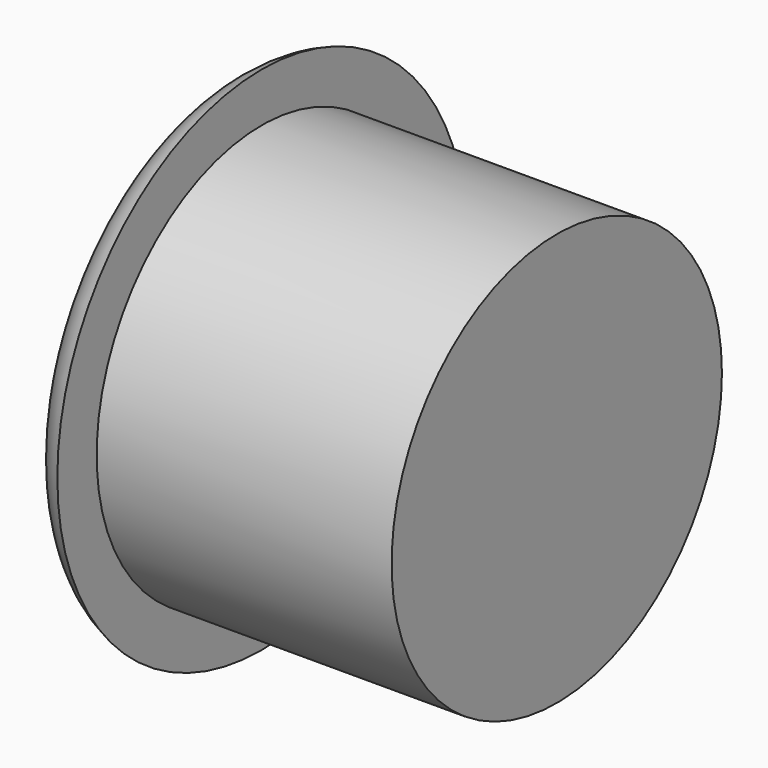
from build123d import *

# Parameters (mm, degrees)
F1_R     = 10.5
F2_DEPTH = 15
F3_R     = 13
F4_DEPTH = 2


# Not quite as in the source:
# - a fillet or chamfer that OpenCascade refuses, or shapes differently, is made with other operations: its cross-section is extruded or revolved along the edge and cut away or added


with BuildPart() as f2:
    # F1 (on face) → F2 (new body)
    with BuildSketch(Plane.YZ):
        Circle(F1_R)
    extrude(amount=F2_DEPTH)

    # F3 (on face) → F4 (join)
    with BuildSketch(Plane.YZ):
        Circle(F3_R)
    extrude(amount=-F4_DEPTH)

    # F5: fillet of radius 3 on 1 edges, made by hand

    # F5_s1 → F5_t2 (revolve, cut)
    with BuildSketch(Plane.XY):
        with BuildLine():
            ThreePointArc((0, 13), (-1.4494897428, 11.9036236828), (-2, 10.1715728753))
            Line((-2, 10.1715728753), (-2, 13))
            Line((-2, 13), (0, 13))
        make_face()
    revolve(axis=Axis((-2, 0, 0), (1, 0, 0)), mode=Mode.SUBTRACT)


solid = f2.part
